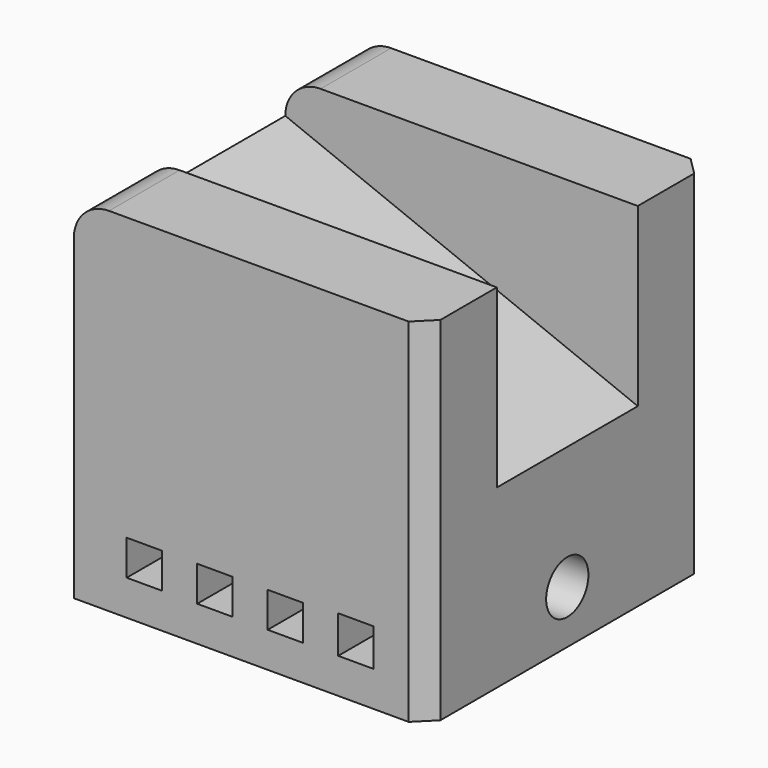
from build123d import *

# Parameters (mm, degrees)
F0_W     = 5
F0_H     = 100
F0_W_2   = 50
F0_H_2   = 40
F1_DEPTH = 100
F2_W     = 10
F2_H     = 10
F2_H_2   = 10.6422880292
F3_DEPTH = 20
F4_R     = 10
F5_R     = 10
F6_SIZE  = 5
F7_SIZE  = 5
F8_SIZE2 = 39.99999
F8_SIZE  = 99.99999


# Not quite as in the source:
# - a fillet or chamfer is up to 0.001 mm smaller than in the source, because OpenCascade refuses the exact size


with BuildPart() as f1:
    # F0 (on Right) → F1 (new body)
    with BuildSketch(Plane.YZ):
        with Locations((2.5, 50)):
            Rectangle(F0_W, F0_H)
        Polygon((5, 100), (5, 0), (50, 0), (95, 0), (95, 100), (75, 100), (75, 90), (75, 50), (25, 50), (25, 90), (25, 100), align=None)
        with BuildLine():
            ThreePointArc((57.5, 15), (55.3033008589, 9.6966991411), (50, 7.5))
            ThreePointArc((50, 7.5), (44.6966991411, 20.3033008589), (57.5, 15))
        make_face(mode=Mode.SUBTRACT)
        with Locations((97.5, 50)):
            Rectangle(F0_W, F0_H)
        with Locations((50, 70)):
            Rectangle(F0_W_2, F0_H_2)
    extrude(amount=-F1_DEPTH)

    # F2 (on Front) → F3 (cut)
    with BuildSketch(Plane.XZ):
        with Locations((-80, 15)):
            Rectangle(F2_W, F2_H)
        with Locations((-60, 15)):
            Rectangle(F2_W, F2_H)
        with Locations((-40, 15)):
            Rectangle(F2_W, F2_H)
        with Locations((-20, 15.3211440146)):
            Rectangle(F2_W, F2_H_2)
    extrude(amount=-F3_DEPTH, mode=Mode.SUBTRACT)

    # F4
    f4_edges = [f1.edges().sort_by_distance(p)[0] for p in [
        (-100, 12.5, 100),
    ]]
    fillet(f4_edges, radius=F4_R)

    # F5
    f5_edges = [f1.edges().sort_by_distance(p)[0] for p in [
        (-100, 87.5, 100),
    ]]
    fillet(f5_edges, radius=F5_R)

    # F6
    f6_edges = [f1.edges().sort_by_distance(p)[0] for p in [
        (0, 0, 50),
    ]]
    chamfer(f6_edges, length=F6_SIZE)

    # F7
    f7_edges = [f1.edges().sort_by_distance(p)[0] for p in [
        (0, 100, 50),
    ]]
    chamfer(f7_edges, length=F7_SIZE)

    # F8 (size 100 and 40 in the source; OpenCascade refuses exactly that, so slightly less here)
    f8_edges = [f1.edges().sort_by_distance(p)[0] for p in [
        (0, 50, 90),
    ]]
    f8_side = f1.faces().sort_by_distance((-50, 50, 90))[0]
    chamfer(f8_edges, length=F8_SIZE, length2=F8_SIZE2, reference=f8_side)


with BuildPart() as f1_1:
    # F9: moved
    add(f1.part.moved(Location((100, 0, 0))))


solid = f1_1.part
